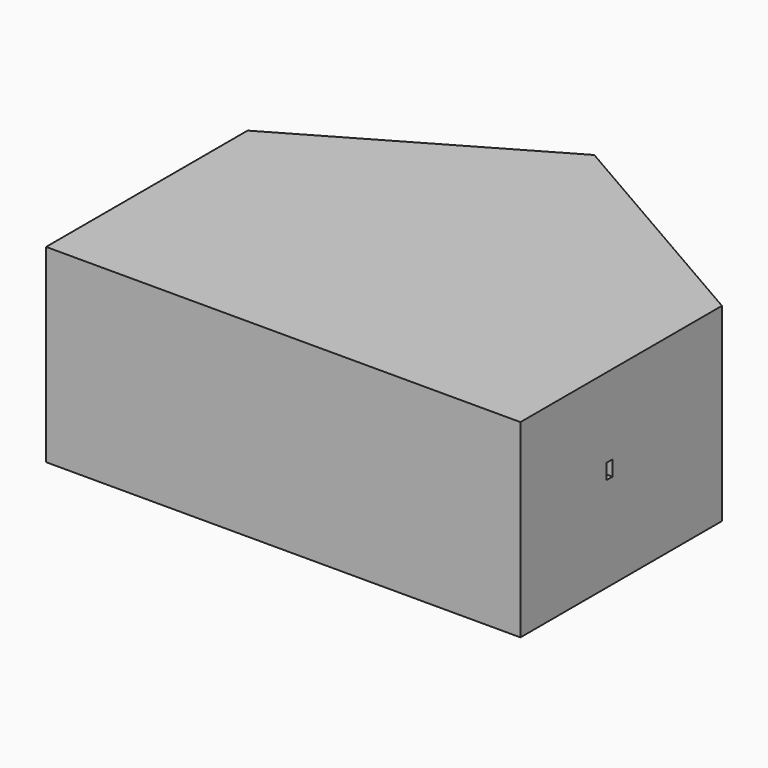
from build123d import *

# Parameters (mm, degrees)
F0_W     = 24.15
F0_H     = 11.7
F1_DEPTH = 9.65
F2_W     = 0.775
F2_H     = 1.55
F3_DEPTH = 48.3
F4_W     = 1.55
F4_H     = 1.55
F5_DEPTH = 10
F6_W     = 1.55
F6_H     = 1.55
F7_DEPTH = 10


with BuildPart() as f1:
    # F0 (on Top) → F1 (new body, symmetric)
    with BuildSketch(Plane.XY):
        Polygon((-24.15, 11.7), (0, 11.7), (-12.075, 32.6145135014), (-24.15, 25.6430090009), align=None)
        with Locations((-12.075, 5.85)):
            Rectangle(F0_W, F0_H)
        with Locations((12.075, 5.85)):
            Rectangle(F0_W, F0_H)
        Polygon((12.075, 32.6145135014), (0, 11.7), (24.15, 11.7), (24.15, 25.6430090009), align=None)
        Polygon((-12.075, 32.6145135014), (0, 11.7), (12.075, 32.6145135014), (0, 39.5860180019), align=None)
    extrude(amount=F1_DEPTH, both=True)

    # F2 (on face) → F3 (cut)
    with BuildSketch(Plane(origin=(-24.15, 0, 0), x_dir=(0, -1, 0), z_dir=(-1, 0, 0))):
        with Locations((-11.3125, 0.775)):
            Rectangle(F2_W, F2_H)
    extrude(amount=-F3_DEPTH, mode=Mode.SUBTRACT)

    # F4 (on face) → F5 (cut)
    with BuildSketch(Plane(origin=(17.1412486121, 29.6895135014, 0), x_dir=(-0.8660254038, 0.5, 0), z_dir=(0.5, 0.8660254038, 0))):
        with Locations((5.85, 0.775)):
            Rectangle(F4_W, F4_H)
        with Locations((5.85, -0.775)):
            Rectangle(F4_W, F4_H)
    extrude(amount=-F5_DEPTH, mode=Mode.SUBTRACT)

    # F6 (on face) → F7 (cut)
    with BuildSketch(Plane(origin=(-17.1412486121, 29.6895135014, 0), x_dir=(-0.8660254038, -0.5, 0), z_dir=(-0.5, 0.8660254038, 0))):
        with Locations((-5.85, -0.775)):
            Rectangle(F6_W, F6_H)
        with Locations((-5.85, 0.775)):
            Rectangle(F6_W, F6_H)
    extrude(amount=-F7_DEPTH, mode=Mode.SUBTRACT)


solid = f1.part
